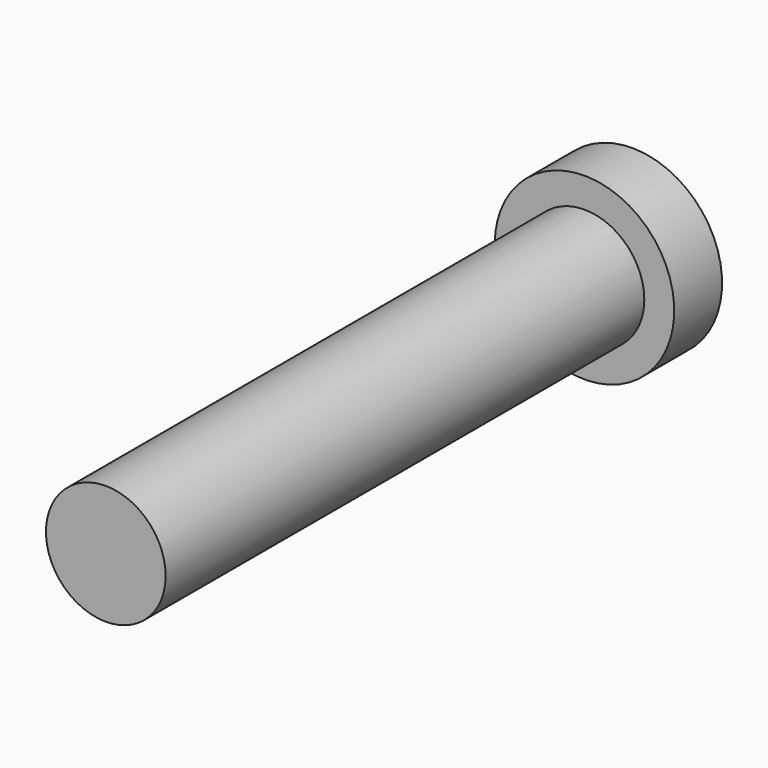
from build123d import *

# Parameters (mm, degrees)
F0_R     = 12.7
F1_DEPTH = 127
F2_R     = 19.05
F2_R_2   = 12.7
F3_DEPTH = 12.7


with BuildPart() as f1:
    # F0 (on Front) → F1 (new body)
    with BuildSketch(Plane.XZ):
        Circle(F0_R)
    extrude(amount=F1_DEPTH)

    # F2 (on face) → F3 (join)
    with BuildSketch(Plane(origin=(0, 0, 0), x_dir=(-1, 0, 0), z_dir=(0, 1, 0))):
        Circle(F2_R)
        Circle(F2_R_2, mode=Mode.SUBTRACT)
        Circle(F2_R_2)
    extrude(amount=F3_DEPTH)


solid = f1.part
